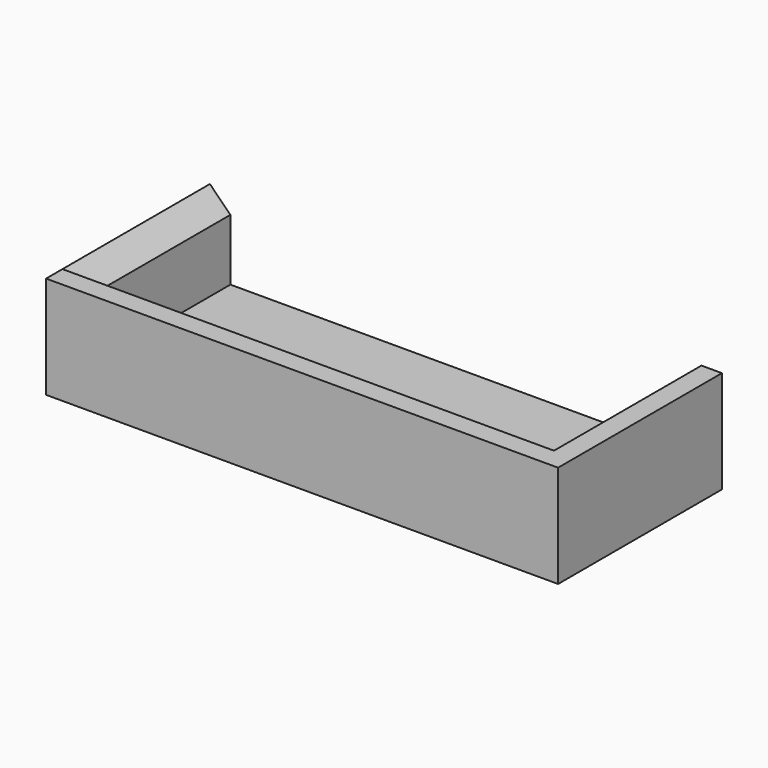
from build123d import *

# Parameters (mm, degrees)
F0_W     = 125
F0_H     = 50
F1_DEPTH = 25
F2_T     = -5
F3_SIZE  = 4.99999


# Not quite as in the source:
# - a fillet or chamfer is up to 0.001 mm smaller than in the source, because OpenCascade refuses the exact size


with BuildPart() as f1:
    # F0 (on Top) → F1 (new body)
    with BuildSketch(Plane.XY):
        with Locations((62.5, 25)):
            Rectangle(F0_W, F0_H)
    extrude(amount=F1_DEPTH)

    # F2
    f2_openings = [f1.faces().sort_by_distance(p)[0] for p in [
        (62.5, 25, 25),
        (62.5, 50, 12.5),
    ]]
    offset(amount=F2_T, openings=f2_openings)

    # F3 (size 5 in the source; OpenCascade refuses exactly that, so slightly less here)
    f3_edges = [f1.edges().sort_by_distance(p)[0] for p in [
        (5, 27.5, 25),
    ]]
    chamfer(f3_edges, length=F3_SIZE)


solid = f1.part
